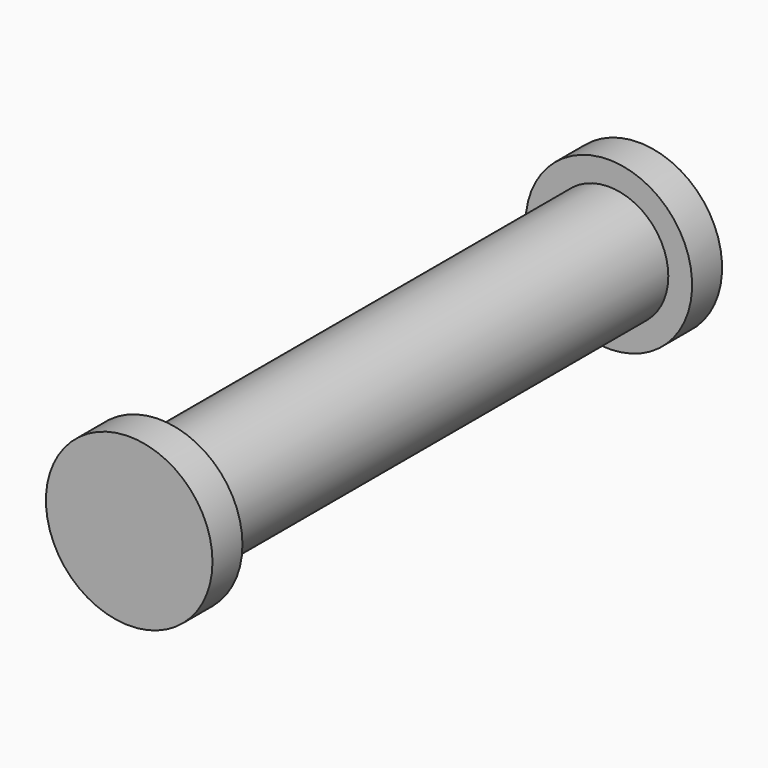
from build123d import *

# Parameters (mm, degrees)
F0_R      = 3.175
F1_DEPTH  = 10
F1_FACE_R = 3.175
F2_R      = 4.445
F3_DEPTH  = 2
F4_DEPTH  = 20
F5_R      = 4.445
F6_DEPTH  = 2


with BuildPart() as f1:
    # F0 (on Front) → F1 (new body)
    with BuildSketch(Plane.XZ):
        with Locations((-68.0588558316, 31.7334979773)):
            Circle(F0_R)
    extrude(amount=F1_DEPTH)

    # F1_face (on face) + F2 (on face) → F3 (join)
    with BuildSketch(Plane(origin=(-68.0588558316, -10, 31.7334979773), x_dir=(1, 0, 0), z_dir=(0, -1, 0))):
        Circle(F1_FACE_R)
    with BuildSketch(Plane.XZ.offset(10)):
        with Locations((-68.0588558316, 31.7334979773)):
            Circle(F2_R)
    extrude(amount=F3_DEPTH)

    # F4 (add): a face of the model
    f4_faces = [f1.faces().sort_by_distance(p)[0] for p in [
        (-68.0588558316, 0, 31.7334979773),
    ]]
    extrude(f4_faces, amount=F4_DEPTH)

    # F5 (on face) → F6 (join)
    with BuildSketch(Plane(origin=(0, 20, 0), x_dir=(-1, 0, 0), z_dir=(0, 1, 0))):
        with Locations((68.0588558316, 31.7334979773)):
            Circle(F5_R)
    extrude(amount=F6_DEPTH)


solid = f1.part
